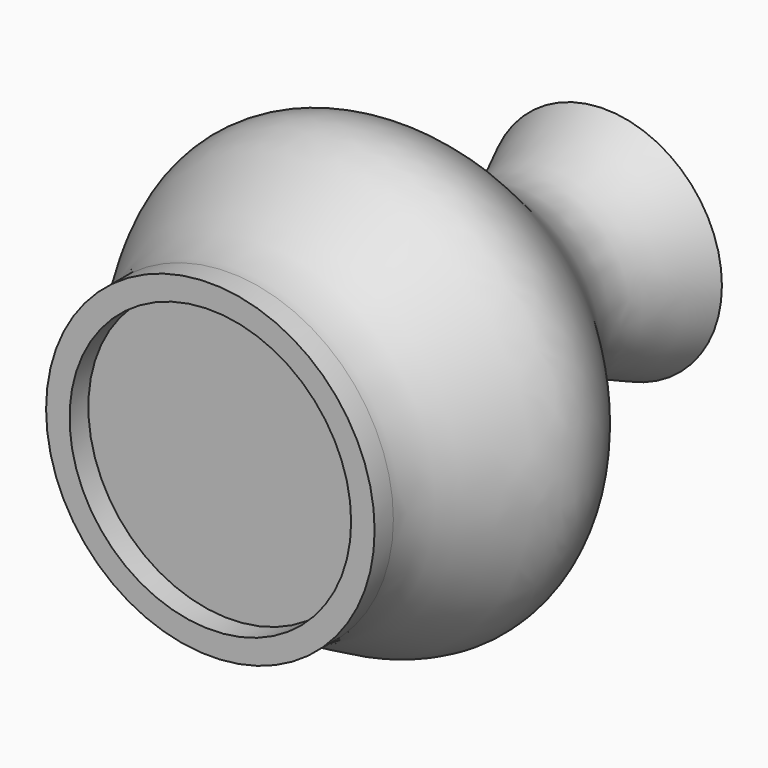
from build123d import *

# Parameters (mm, degrees)
F2_T = 2


# Not quite as in the source:
# - a shell that OpenCascade refuses in one call is made with other operations: the cavity is built on its own and cut out


with BuildPart() as f1:
    # F0 (on Top) → F1 (revolve)
    with BuildSketch(Plane.XY):
        with BuildLine():
            add(Edge.make_bspline(
                [(25, 80.1909700036), (21.3941747588, 72.6824155929), (14.9084310427, 57.4422037156), (33.1888057684, 38.7824688485), (58.1779709373, 13.3224245963), (34.3693904579, -8.2805072889), (35, -19.8090299964)],
                knots=[0, 0, 0, 0, 0.2247709599, 0.4593972663, 0.716316281, 1, 1, 1, 1], degree=3))
            Line((25, 80.1909700036), (0, 80.1909700036))
            Line((0, 80.1909700036), (0, -19.8090299964))
            Line((0, -19.8090299964), (30, -19.8090299964))
            Line((30, -19.8090299964), (30, -24.8090299964))
            Line((30, -24.8090299964), (35, -24.8090299964))
            Line((35, -24.8090299964), (35, -19.8090299964))
        make_face()
    revolve(axis=Axis((0, 30.1909700036, 0), (0, -1, 0)))

    # F2: shell of thickness 2, made by hand


with BuildPart() as f2_core1:
    # F2_t2: copy of F1
    add(f1.part)

    # the walls: a layer under each face that stays
    f2_faces = [f2_core1.faces().sort_by_distance(p)[0] for p in [
        (-36.8980626212, 34.9663384335, 0),
        (-35, -22.3090299964, 0),
        (23.3333333333, -24.8090299964, -23.3333333333),
        (-30, -22.3090299964, 0),
        (0, -19.8090299964, 0),
    ]]
    thicken(f2_faces, amount=-F2_T, mode=Mode.SUBTRACT)

    # F2_s3 → F2_t4 (revolve, cut)
    with BuildSketch(Plane.XY):
        Polygon((29.98, -19.8290299964), (32, -19.8090299964), (32, -17.8090299964), (30, -17.8090299964), align=None)
    revolve(axis=Axis((0, -19.8090299964, 0), (0, -1, 0)), mode=Mode.SUBTRACT)


with BuildPart() as f1_1:
    add(f1.part)

    # what is left inside the walls is the cavity
    f2_cavity = [f2_core1.part.solids().sort_by_distance(p)[0] for p in [
        (-22.512298, 47.591043, 0),
    ]]
    add(f2_cavity, mode=Mode.SUBTRACT)


solid = f1_1.part
